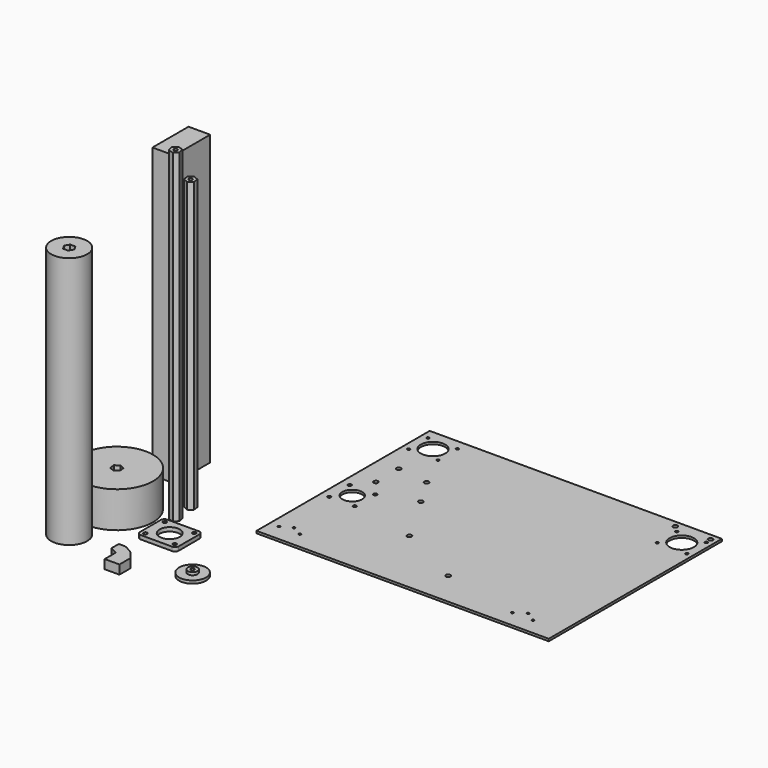
from build123d import *

# Parameters (mm, degrees)
F1_R      = 50.8
F2_DEPTH  = 50.8
F1_R_2    = 2.5527
F3_DEPTH  = 457.2
F4_DEPTH  = 406.4
F5_W      = 30.48
F5_H      = 63.5
F6_DEPTH  = 406.4
F5_W_2    = 411.48
F5_H_2    = 304.8
F5_R      = 1.651
F5_R_2    = 2.413
F5_R_3    = 13.97
F5_R_4    = 3.175
F5_R_5    = 1.905
F5_R_6    = 17.145
F7_DEPTH  = 3.175
F8_W      = 54.61
F8_H      = 46.99
F8_R      = 2.54
F8_R_2    = 14.2875
F9_DEPTH  = 5.5
F10_R     = 5.08
F1_R_3    = 25.4
F11_DEPTH = 355.6
F13_DEPTH = 12.7
F14_R     = 19.05
F14_R_2   = 6.875
F15_DEPTH = 4.064
F14_R_3   = 2.4765
F16_DEPTH = 8.0391


# Not quite as in the source:
# - a length typed as a fraction of an inch, garbled in the dataset ("3 / 203.2 mm" for 3/8 in), is restored


with BuildPart() as f2:
    # F1 (on Top) → F2 (new body)
    with BuildSketch(Plane.XY):
        with Locations((-143.5220688581, 65.6463503838)):
            Circle(F1_R)
        Polygon((-137.5822819568, 70.0230345219), (-136.7618557595, 62.6906861032), (-142.7016426608, 58.3140019651), (-149.4618557595, 61.2696662456), (-150.2822819568, 68.6020146643), (-144.3424950555, 72.9786988025), align=None, mode=Mode.SUBTRACT)
    extrude(amount=F2_DEPTH)


with BuildPart() as f3:
    # F1 (on Top) → F3 (new body)
    with BuildSketch(Plane.XY):
        Polygon((-76.9374659596, 80.7480279679), (-71.5035152941, 86.0008461668), (-73.3356139631, 93.3331945856), (-80.6016632976, 95.4127248054), (-86.0356139631, 90.1599066064), (-84.2035152941, 82.8275581877), align=None)
        with Locations((-78.7695646286, 88.0803763866)):
            Circle(F1_R_2, mode=Mode.SUBTRACT)
    extrude(amount=F3_DEPTH)


with BuildPart() as f4:
    # F1 (on Top) → F4 (new body)
    with BuildSketch(Plane.XY):
        Polygon((-76.1031942211, 116.8783073278), (-77.011935655, 124.2106557465), (-83.816306372, 127.0898367887), (-89.711935655, 122.636669412), (-88.8031942211, 115.3043209933), (-81.9988235041, 112.4251399512), align=None)
        with Locations((-82.9075649381, 119.7574883699)):
            Circle(F1_R_2, mode=Mode.SUBTRACT)
    extrude(amount=F4_DEPTH)


with BuildPart() as f6:
    # F5 (on Top) → F6 (new body)
    with BuildSketch(Plane.XY):
        with Locations((-147.7291895056, 184.2925612926)):
            Rectangle(F5_W, F5_H)
    extrude(amount=F6_DEPTH)


with BuildPart() as f7:
    # F5 (on Top) → F7 (new body)
    with BuildSketch(Plane.XY):
        with Locations((218.4401935768, 268.5065377951)):
            Rectangle(F5_W_2, F5_H_2)
        with Locations((25.7042471561, 139.6628220876)):
            Circle(F5_R, mode=Mode.SUBTRACT)
        with Locations((54.9030725154, 139.6628220876)):
            Circle(F5_R, mode=Mode.SUBTRACT)
        with Locations((40.3065336868, 147.7002253135)):
            Circle(F5_R, mode=Mode.SUBTRACT)
        with Locations((24.5749604191, 229.3479357149)):
            Circle(F5_R_2, mode=Mode.SUBTRACT)
        with Locations((60.4959849034, 229.3479357149)):
            Circle(F5_R_2, mode=Mode.SUBTRACT)
        with Locations((42.5354726613, 247.308447957)):
            Circle(F5_R_3, mode=Mode.SUBTRACT)
        with Locations((24.5749604191, 265.2689601992)):
            Circle(F5_R_2, mode=Mode.SUBTRACT)
        with Locations((60.4959849034, 265.2689601992)):
            Circle(F5_R_2, mode=Mode.SUBTRACT)
        with Locations((244.0686225891, 164.1625314951)):
            Circle(F5_R_4, mode=Mode.SUBTRACT)
        with Locations((354.0593478829, 139.6628220876)):
            Circle(F5_R, mode=Mode.SUBTRACT)
        with Locations((383.2581732422, 139.6628220876)):
            Circle(F5_R, mode=Mode.SUBTRACT)
        with Locations((368.6587605625, 149.0740080674)):
            Circle(F5_R, mode=Mode.SUBTRACT)
        with Locations((151.46702528, 211.7215096951)):
            Circle(F5_R_4, mode=Mode.SUBTRACT)
        with Locations((42.5354726613, 288.8645529747)):
            Circle(F5_R_4, mode=Mode.SUBTRACT)
        with Locations((110.3709191084, 283.2107245922)):
            Circle(F5_R_4, mode=Mode.SUBTRACT)
        with Locations((42.5354726613, 329.2627334595)):
            Circle(F5_R_4, mode=Mode.SUBTRACT)
        with Locations((86.6077169776, 323.1149613857)):
            Circle(F5_R_4, mode=Mode.SUBTRACT)
        with Locations((21.7963726613, 372.3605266151)):
            Circle(F5_R_5, mode=Mode.SUBTRACT)
        with Locations((63.2745726613, 372.3605266151)):
            Circle(F5_R_5, mode=Mode.SUBTRACT)
        with Locations((42.5354726613, 389.4420266151)):
            Circle(F5_R_6, mode=Mode.SUBTRACT)
        with Locations((21.7963726613, 406.5235266151)):
            Circle(F5_R_5, mode=Mode.SUBTRACT)
        with Locations((63.2745726613, 406.5235266151)):
            Circle(F5_R_5, mode=Mode.SUBTRACT)
        with Locations((374.5998525414, 369.1934934196)):
            Circle(F5_R_5, mode=Mode.SUBTRACT)
        with Locations((416.0780525414, 369.1934934196)):
            Circle(F5_R_5, mode=Mode.SUBTRACT)
        with Locations((395.3389525414, 386.2749934196)):
            Circle(F5_R_6, mode=Mode.SUBTRACT)
        with Locations((374.5998525414, 403.3564934196)):
            Circle(F5_R_5, mode=Mode.SUBTRACT)
        with Locations((365.6701743603, 412.1054336176)):
            Circle(F5_R_4, mode=Mode.SUBTRACT)
        with Locations((416.0780525414, 403.3564934196)):
            Circle(F5_R_5, mode=Mode.SUBTRACT)
        with Locations((415.2901935768, 412.1054336176)):
            Circle(F5_R_4, mode=Mode.SUBTRACT)
    extrude(amount=F7_DEPTH)


with BuildPart() as f9:
    # F8 (on Top) → F9 (new body)
    with BuildSketch(Plane.XY):
        with Locations((-55.5882994086, 48.7068889356)):
            Rectangle(F8_W, F8_H)
        with Locations((-76.3242393732, 31.6212321949)):
            Circle(F8_R, mode=Mode.SUBTRACT)
        with Locations((-34.8523594439, 31.6212321949)):
            Circle(F8_R, mode=Mode.SUBTRACT)
        with Locations((-76.3242393732, 65.7925456762)):
            Circle(F8_R, mode=Mode.SUBTRACT)
        with Locations((-55.5882994086, 48.7068889356)):
            Circle(F8_R_2, mode=Mode.SUBTRACT)
        with Locations((-34.8523594439, 65.7925456762)):
            Circle(F8_R, mode=Mode.SUBTRACT)
    extrude(amount=F9_DEPTH)

    # F10
    f10_edges = [f9.edges().sort_by_distance(p)[0] for p in [
        (-28.283299, 25.211889, 2.75),
        (-82.893299, 25.211889, 2.75),
        (-28.283299, 72.201889, 2.75),
        (-82.893299, 72.201889, 2.75),
    ]]
    fillet(f10_edges, radius=F10_R)


with BuildPart() as f11:
    # F1 (on Top) → F11 (new body)
    with BuildSketch(Plane.XY):
        with Locations((-146.5940475464, -14.5036224276)):
            Circle(F1_R_3)
        Polygon((-139.2616991277, -14.5036224276), (-142.927873337, -20.8536224276), (-150.2602217557, -20.8536224276), (-153.9263959651, -14.5036224276), (-150.2602217557, -8.1536224276), (-142.927873337, -8.1536224276), align=None, mode=Mode.SUBTRACT)
    extrude(amount=F11_DEPTH)


with BuildPart() as f13:
    # F12 (on Top) → F13 (new body)
    with BuildSketch(Plane.XY):
        with BuildLine():
            Line((-74.5646499772, -29.8816310388), (-64.2275132914, -35.5503847969))
            Line((-64.2275132914, -35.5503847969), (-64.2275132914, -54.8908366037))
            Line((-64.2275132914, -54.8908366037), (-43.5339800427, -54.8908366037))
            Line((-43.5339800427, -54.8908366037), (-43.5339800427, -35.6788924437))
            Line((-43.5339800427, -35.6788924437), (-50.785745993, -26.3120287944))
            ThreePointArc((-50.785745993, -26.3120287944), (-52.4432251073, -24.5479385551), (-54.4052992591, -23.1303644266))
            Line((-54.4052992591, -23.1303644266), (-61.5296247054, -18.9540358114))
            ThreePointArc((-61.5296247054, -18.9540358114), (-64.6246922895, -17.6539842457), (-67.9522622434, -17.2103000951))
            Line((-67.9522622434, -17.2103000951), (-74.5646499772, -17.2103000951))
            Line((-74.5646499772, -17.2103000951), (-74.5646499772, -29.8816310388))
        make_face()
    extrude(amount=F13_DEPTH)


with BuildPart() as f15:
    # F14 (on Top) → F15 (new body)
    with BuildSketch(Plane.XY):
        with Locations((20.855544135, -6.5172538161)):
            Circle(F14_R)
        with Locations((20.855544135, -6.5172538161)):
            Circle(F14_R_2, mode=Mode.SUBTRACT)
    extrude(amount=F15_DEPTH)

    # F14 (on Top) → F16 (join)
    with BuildSketch(Plane.XY):
        with Locations((20.855544135, -6.5172538161)):
            Circle(F14_R_2)
        with Locations((20.855544135, -6.5172538161)):
            Circle(F14_R_3, mode=Mode.SUBTRACT)
    extrude(amount=F16_DEPTH)


solid = Compound([f2.part, f3.part, f4.part, f6.part, f7.part, f9.part, f11.part, f13.part, f15.part])
